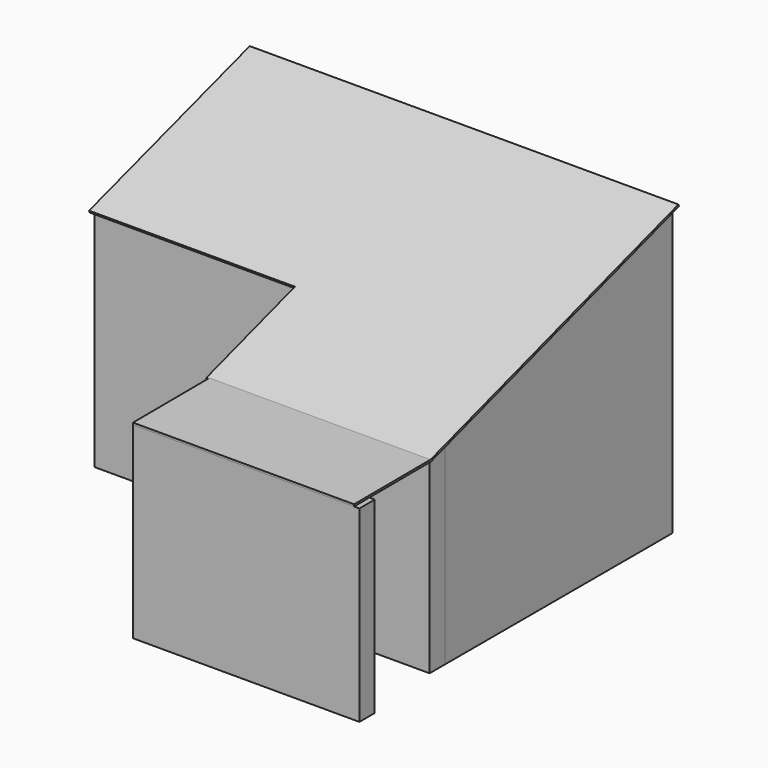
from build123d import *

# Parameters (mm, degrees)
F8_DEPTH  = 3600
F10_DEPTH = 3740
F11_W     = 925
F11_H     = 1560
F12_DEPTH = 3560
F13_DEPTH = 25
F16_DEPTH = 25
F1_W      = 598.0567009747
F1_H      = 600
F17_DEPTH = 10
F1_W_2    = 600
F1_H_2    = 289.0001684427
F1_H_3    = 289.0002566576
F1_W_3    = 432.8018852323
F1_H_4    = 449.4931197166
F1_H_5    = 288.5067301989
F1_H_6    = 449.4932079315
F1_H_7    = 288.506641984
F1_H_8    = 448.8179183006
F1_H_9    = 289.1819316149
F1_W_4    = 564.9999634922
F1_H_10   = 448.8180065155
F18_W     = 2781.1407826908
F18_H     = 1203.9378546259
F19_DEPTH = 25


# Not quite as in the source:
# - ends of sketch curves that miss each other by under 0.0002 mm in the source are joined


with BuildPart() as f8:
    # F2 (on face) → F8 (new body)
    with BuildSketch(Plane.XY):
        Polygon((2415.198802948, 906.08273983), (-2414.801197052, 906.08273983), (-2414.801197052, 666.0830950737), (2415.1981146634, 666.0830950737), (2415.1981146634, 666.08273983), (2415.198802948, 666.08273983), align=None)
    extrude(amount=F8_DEPTH)


with BuildPart() as f8b:
    # F3 (on face) → F8, piece 2 (new body)
    with BuildSketch(Plane.XY):
        Polygon((2655.1978492737, -2673.7489271164), (2655.1978492737, 906.2510728836), (2415.1978492737, 906.2510728836), (2415.1978492737, 666.0830950737), (2415.1981146634, 666.0830950737), (2415.1981146634, -2673.7489271164), align=None)
    extrude(amount=F8_DEPTH)


with BuildPart() as f8c:
    # F4 (on Top) → F8, piece 3 (new body)
    with BuildSketch(Plane.XY):
        Polygon((-2415.9480808742, -1303.9169322286), (-2416.0007220573, 906.0485089984), (-2655.9480808742, 906.0427934733), (-2655.9480808742, -1303.9169322286), align=None)
    extrude(amount=F8_DEPTH)


with BuildPart() as f8d:
    # F5 (on Top) → F8, piece 4 (new body)
    with BuildSketch(Plane.XY):
        Polygon((-2655.9605169296, -1543.9375956409), (154.0394830704, -1543.9378023148), (154.0394830704, -1303.9378023148), (-2655.9605169296, -1303.9378023148), align=None)
    extrude(amount=F8_DEPTH)


with BuildPart() as f8e:
    # F6 (on Top) → F8, piece 5 (new body)
    with BuildSketch(Plane.XY):
        Polygon((155.0143378906, -1303.8981531892), (-84.9330209262, -1303.9038687143), (-84.9330209262, -3911.8513970537), (-84.9387364513, -3911.8513971899), (-84.9330209262, -4151.7987560067), (2762.9618663663, -4151.7987560067), (2762.9618663663, -3911.7835604471), (155.0764589722, -3911.8456800489), align=None)
    extrude(amount=F8_DEPTH)


with BuildPart() as f8f:
    # F7 (on Top) → F8, piece 6 (new body)
    with BuildSketch(Plane.XY):
        Polygon((1415.1374530792, -2913.7420082092), (2655.1374530792, -2913.7423634529), (2655.1374530792, -2673.7423634529), (1415.1374530792, -2673.7423634529), align=None)
    extrude(amount=F8_DEPTH)


with BuildPart() as f10_tool:
    # F9 (on Right) → F10 (new body, symmetric)
    with BuildSketch(Plane.YZ):
        Polygon((-4392.7998542786, 2362.4069690704), (-2947.8775242662, 2370), (987.2349500656, 3623.4698295593), (987.2349500656, 4423.1357574463), (-4372.3435401917, 4418.2653427124), align=None)
    extrude(amount=F10_DEPTH, both=True)


with BuildPart() as f8_1:
    add(f8.part)

    # F10: cut by f10_tool
    add(f10_tool.part, mode=Mode.SUBTRACT)


with BuildPart() as f8b_1:
    add(f8b.part)

    # F10: cut by f10_tool
    add(f10_tool.part, mode=Mode.SUBTRACT)


with BuildPart() as f8c_1:
    add(f8c.part)

    # F10: cut by f10_tool
    add(f10_tool.part, mode=Mode.SUBTRACT)

    # F11 (on Right) → F12 (cut)
    with BuildSketch(Plane.YZ):
        with Locations((-165.287232399, 1705.6165027618)):
            Rectangle(F11_W, F11_H)
    extrude(amount=-F12_DEPTH, mode=Mode.SUBTRACT)


with BuildPart() as f8d_1:
    add(f8d.part)

    # F10: cut by f10_tool
    add(f10_tool.part, mode=Mode.SUBTRACT)


with BuildPart() as f8e_1:
    add(f8e.part)

    # F10: cut by f10_tool
    add(f10_tool.part, mode=Mode.SUBTRACT)


with BuildPart() as f8f_1:
    add(f8f.part)

    # F10: cut by f10_tool
    add(f10_tool.part, mode=Mode.SUBTRACT)


with BuildPart() as f13:
    # F0 (on Top) → F13 (new body)
    with BuildSketch(Plane.XY):
        Polygon((2415.1981146634, 666.0830950737), (-2414.8018853366, 666.0830950737), (-2414.8018853366, -1303.9169049263), (155.1981146634, -1303.9169049263), (155.1981146634, -2673.9169049263), (587.9999998957, -2673.9169049263), (596.9996098429, -2673.9169049263), (1196.9996098429, -2673.9169049263), (1208.1418037415, -2673.9169049263), (1808.1418037415, -2673.9168167114), (1817.1414136887, -2673.9169049263), (2415.1981146634, -2673.9169049263), align=None)
    extrude(amount=F13_DEPTH)


with BuildPart() as f16:
    # F15 (on offset) → F16 (new body)
    with BuildSketch(Plane(origin=(0, -956.9367245377, 3004.1837091511), x_dir=(1, 0, 0), z_dir=(0, -0.3035089574, 0.9528285852))):
        Polygon((2697.4198818207, 2005.6664943695), (-2695.618391037, 2005.6664943695), (-2702.8093338013, -635.6807947159), (-114.1507923603, -635.6807947159), (-114.1507923603, -2099.74193573), (2697.4198818207, -2099.74193573), align=None)
    extrude(amount=F16_DEPTH)

    # F18 (on face) → F19 (join)
    with BuildSketch(Plane(origin=(0, -12.5353498726, 2385.4251501663), x_dir=(1, 0, 0), z_dir=(0, -0.0052549026, 0.9999861929))):
        with Locations((1305.6373704191, -3537.3516308172)):
            Rectangle(F18_W, F18_H)
    extrude(amount=F19_DEPTH)


with BuildPart() as f17:
    # F1 (on Top) → F17 (new body)
    with BuildSketch(Plane.XY):
        with Locations((2115.828159675, -2373.4318685532)):
            Rectangle(F1_W, F1_H)
    extrude(amount=F17_DEPTH)


with BuildPart() as f17b:
    # F1 (on Top) → F17, piece 2 (new body)
    with BuildSketch(Plane.XY):
        with Locations((2115.828159675, -1761.4317917824)):
            Rectangle(F1_W, F1_H)
    extrude(amount=F17_DEPTH)


with BuildPart() as f17c:
    # F1 (on Top) → F17, piece 3 (new body)
    with BuildSketch(Plane.XY):
        with Locations((2115.828159675, -1154.4322752953)):
            Rectangle(F1_W, F1_H)
    extrude(amount=F17_DEPTH)


with BuildPart() as f17d:
    # F1 (on Top) → F17, piece 4 (new body)
    with BuildSketch(Plane.XY):
        with Locations((2115.828159675, -542.4321985245)):
            Rectangle(F1_W, F1_H)
    extrude(amount=F17_DEPTH)


with BuildPart() as f17e:
    # F1 (on Top) → F17, piece 5 (new body)
    with BuildSketch(Plane.XY):
        with Locations((2115.828159675, 65.5677980185)):
            Rectangle(F1_W, F1_H)
    extrude(amount=F17_DEPTH)


with BuildPart() as f17f:
    # F1 (on Top) → F17, piece 6 (new body)
    with BuildSketch(Plane.XY):
        Polygon((1816.7998091877, 666.5681314468), (1816.7998091877, 377.5678747892), (2414.8565101624, 377.5678747892), (2411.5405082703, 666.5681314468), align=None)
    extrude(amount=F17_DEPTH)


with BuildPart() as f17g:
    # F1 (on Top) → F17, piece 7 (new body)
    with BuildSketch(Plane.XY):
        with Locations((1507.8001992404, -2373.4317803383)):
            Rectangle(F1_W_2, F1_H)
    extrude(amount=F17_DEPTH)


with BuildPart() as f17h:
    # F1 (on Top) → F17, piece 8 (new body)
    with BuildSketch(Plane.XY):
        with Locations((1507.8001992404, -1761.4317035675)):
            Rectangle(F1_W_2, F1_H)
    extrude(amount=F17_DEPTH)


with BuildPart() as f17i:
    # F1 (on Top) → F17, piece 9 (new body)
    with BuildSketch(Plane.XY):
        with Locations((1507.8001992404, -1154.4321870804)):
            Rectangle(F1_W_2, F1_H)
    extrude(amount=F17_DEPTH)


with BuildPart() as f17j:
    # F1 (on Top) → F17, piece 10 (new body)
    with BuildSketch(Plane.XY):
        with Locations((1507.8001992404, -542.4321103096)):
            Rectangle(F1_W_2, F1_H)
    extrude(amount=F17_DEPTH)


with BuildPart() as f17k:
    # F1 (on Top) → F17, piece 11 (new body)
    with BuildSketch(Plane.XY):
        with Locations((1507.8001992404, 65.5678862333)):
            Rectangle(F1_W_2, F1_H)
    extrude(amount=F17_DEPTH)


with BuildPart() as f17l:
    # F1 (on Top) → F17, piece 12 (new body)
    with BuildSketch(Plane.XY):
        with Locations((1507.8001992404, 522.0680472255)):
            Rectangle(F1_W_2, F1_H_2)
    extrude(amount=F17_DEPTH)


with BuildPart() as f17m:
    # F1 (on Top) → F17, piece 13 (new body)
    with BuildSketch(Plane.XY):
        with Locations((896.6580053419, -2373.4318685532)):
            Rectangle(F1_W_2, F1_H)
    extrude(amount=F17_DEPTH)


with BuildPart() as f17n:
    # F1 (on Top) → F17, piece 14 (new body)
    with BuildSketch(Plane.XY):
        with Locations((896.6580053419, -1761.4317917824)):
            Rectangle(F1_W_2, F1_H)
    extrude(amount=F17_DEPTH)


with BuildPart() as f17o:
    # F1 (on Top) → F17, piece 15 (new body)
    with BuildSketch(Plane.XY):
        with Locations((896.6580053419, -1154.4322752953)):
            Rectangle(F1_W_2, F1_H)
    extrude(amount=F17_DEPTH)


with BuildPart() as f17p:
    # F1 (on Top) → F17, piece 16 (new body)
    with BuildSketch(Plane.XY):
        with Locations((896.6580053419, -542.4321985245)):
            Rectangle(F1_W_2, F1_H)
    extrude(amount=F17_DEPTH)


with BuildPart() as f17q:
    # F1 (on Top) → F17, piece 17 (new body)
    with BuildSketch(Plane.XY):
        with Locations((896.6580053419, 65.5677980185)):
            Rectangle(F1_W_2, F1_H)
    extrude(amount=F17_DEPTH)


with BuildPart() as f17r:
    # F1 (on Top) → F17, piece 18 (new body)
    with BuildSketch(Plane.XY):
        with Locations((896.6580053419, 522.068003118)):
            Rectangle(F1_W_2, F1_H_3)
    extrude(amount=F17_DEPTH)


with BuildPart() as f17s:
    # F1 (on Top) → F17, piece 19 (new body)
    with BuildSketch(Plane.XY):
        with Locations((371.2574527785, -2373.4318685532)):
            Rectangle(F1_W_3, F1_H)
    extrude(amount=F17_DEPTH)


with BuildPart() as f17t:
    # F1 (on Top) → F17, piece 20 (new body)
    with BuildSketch(Plane.XY):
        with Locations((371.2574527785, -1761.4317035675)):
            Rectangle(F1_W_3, F1_H)
    extrude(amount=F17_DEPTH)


with BuildPart() as f17u:
    # F1 (on Top) → F17, piece 21 (new body)
    with BuildSketch(Plane.XY):
        Polygon((587.6583953947, -854.4321870804), (-12.3416046053, -854.4321870804), (-12.3416046053, -1303.4318685532), (150.5999565125, -1303.4318685532), (154.8565101624, -1303.4318685532), (154.8565101624, -1454.4321870804), (587.6583953947, -1454.4321870804), align=None)
    extrude(amount=F17_DEPTH)


with BuildPart() as f17v:
    # F1 (on Top) → F17, piece 22 (new body)
    with BuildSketch(Plane.XY):
        with Locations((287.6583953947, -542.4321103096)):
            Rectangle(F1_W_2, F1_H)
    extrude(amount=F17_DEPTH)


with BuildPart() as f17w:
    # F1 (on Top) → F17, piece 23 (new body)
    with BuildSketch(Plane.XY):
        with Locations((287.6583953947, 65.5678862333)):
            Rectangle(F1_W_2, F1_H)
    extrude(amount=F17_DEPTH)


with BuildPart() as f17x:
    # F1 (on Top) → F17, piece 24 (new body)
    with BuildSketch(Plane.XY):
        with Locations((287.6583953947, 522.0680472255)):
            Rectangle(F1_W_2, F1_H_2)
    extrude(amount=F17_DEPTH)


with BuildPart() as f17y:
    # F1 (on Top) → F17, piece 25 (new body)
    with BuildSketch(Plane.XY):
        with Locations((-323.4801514447, -1078.6853086948)):
            Rectangle(F1_W_2, F1_H_4)
    extrude(amount=F17_DEPTH)


with BuildPart() as f17z:
    # F1 (on Top) → F17, piece 26 (new body)
    with BuildSketch(Plane.XY):
        with Locations((-323.4801514447, -541.9386720657)):
            Rectangle(F1_W_2, F1_H)
    extrude(amount=F17_DEPTH)


with BuildPart() as f17ba:
    # F1 (on Top) → F17, piece 27 (new body)
    with BuildSketch(Plane.XY):
        with Locations((-323.4801514447, 66.0613244772)):
            Rectangle(F1_W_2, F1_H)
    extrude(amount=F17_DEPTH)


with BuildPart() as f17bb:
    # F1 (on Top) → F17, piece 28 (new body)
    with BuildSketch(Plane.XY):
        with Locations((-323.4801514447, 522.3147663474)):
            Rectangle(F1_W_2, F1_H_5)
    extrude(amount=F17_DEPTH)


with BuildPart() as f17bc:
    # F1 (on Top) → F17, piece 29 (new body)
    with BuildSketch(Plane.XY):
        with Locations((-932.4797613919, -1078.6852645874)):
            Rectangle(F1_W_2, F1_H_6)
    extrude(amount=F17_DEPTH)


with BuildPart() as f17bd:
    # F1 (on Top) → F17, piece 30 (new body)
    with BuildSketch(Plane.XY):
        with Locations((-932.4797613919, -541.9385838509)):
            Rectangle(F1_W_2, F1_H)
    extrude(amount=F17_DEPTH)


with BuildPart() as f17be:
    # F1 (on Top) → F17, piece 31 (new body)
    with BuildSketch(Plane.XY):
        with Locations((-932.4797613919, 66.0614126921)):
            Rectangle(F1_W_2, F1_H)
    extrude(amount=F17_DEPTH)


with BuildPart() as f17bf:
    # F1 (on Top) → F17, piece 32 (new body)
    with BuildSketch(Plane.XY):
        with Locations((-932.4797613919, 522.3148104548)):
            Rectangle(F1_W_2, F1_H_7)
    extrude(amount=F17_DEPTH)


with BuildPart() as f17bg:
    # F1 (on Top) → F17, piece 33 (new body)
    with BuildSketch(Plane.XY):
        with Locations((-1541.1439163983, -1079.0229094028)):
            Rectangle(F1_W_2, F1_H_8)
    extrude(amount=F17_DEPTH)


with BuildPart() as f17bh:
    # F1 (on Top) → F17, piece 34 (new body)
    with BuildSketch(Plane.XY):
        with Locations((-1541.1439163983, -542.6138734818)):
            Rectangle(F1_W_2, F1_H)
    extrude(amount=F17_DEPTH)


with BuildPart() as f17bi:
    # F1 (on Top) → F17, piece 35 (new body)
    with BuildSketch(Plane.XY):
        with Locations((-1541.1439163983, 65.3861230612)):
            Rectangle(F1_W_2, F1_H)
    extrude(amount=F17_DEPTH)


with BuildPart() as f17bj:
    # F1 (on Top) → F17, piece 36 (new body)
    with BuildSketch(Plane.XY):
        with Locations((-1541.1439163983, 521.9771656394)):
            Rectangle(F1_W_2, F1_H_9)
    extrude(amount=F17_DEPTH)


with BuildPart() as f17bk:
    # F1 (on Top) → F17, piece 37 (new body)
    with BuildSketch(Plane.XY):
        with Locations((-2132.6435080916, -1079.0228652954)):
            Rectangle(F1_W_4, F1_H_10)
    extrude(amount=F17_DEPTH)


with BuildPart() as f17bl:
    # F1 (on Top) → F17, piece 38 (new body)
    with BuildSketch(Plane.XY):
        with Locations((-2132.6435080916, -542.6137852669)):
            Rectangle(F1_W_4, F1_H)
    extrude(amount=F17_DEPTH)


with BuildPart() as f17bm:
    # F1 (on Top) → F17, piece 39 (new body)
    with BuildSketch(Plane.XY):
        with Locations((-2132.6435080916, 65.3862112761)):
            Rectangle(F1_W_4, F1_H)
    extrude(amount=F17_DEPTH)


with BuildPart() as f17bn:
    # F1 (on Top) → F17, piece 40 (new body)
    with BuildSketch(Plane.XY):
        Polygon((-2415.1434898376, 668.9397096634), (-2415.1434898376, 377.3862880468), (-1850.1435263455, 377.3862880468), (-1850.1435263455, 666.5681314468), align=None)
    extrude(amount=F17_DEPTH)


solid = Compound([f8_1.part, f8b_1.part, f8c_1.part, f8d_1.part, f8e_1.part, f8f_1.part, f13.part, f16.part, f17.part, f17b.part, f17c.part, f17d.part, f17e.part, f17f.part, f17g.part, f17h.part, f17i.part, f17j.part, f17k.part, f17l.part, f17m.part, f17n.part, f17o.part, f17p.part, f17q.part, f17r.part, f17s.part, f17t.part, f17u.part, f17v.part, f17w.part, f17x.part, f17y.part, f17z.part, f17ba.part, f17bb.part, f17bc.part, f17bd.part, f17be.part, f17bf.part, f17bg.part, f17bh.part, f17bi.part, f17bj.part, f17bk.part, f17bl.part, f17bm.part, f17bn.part])
